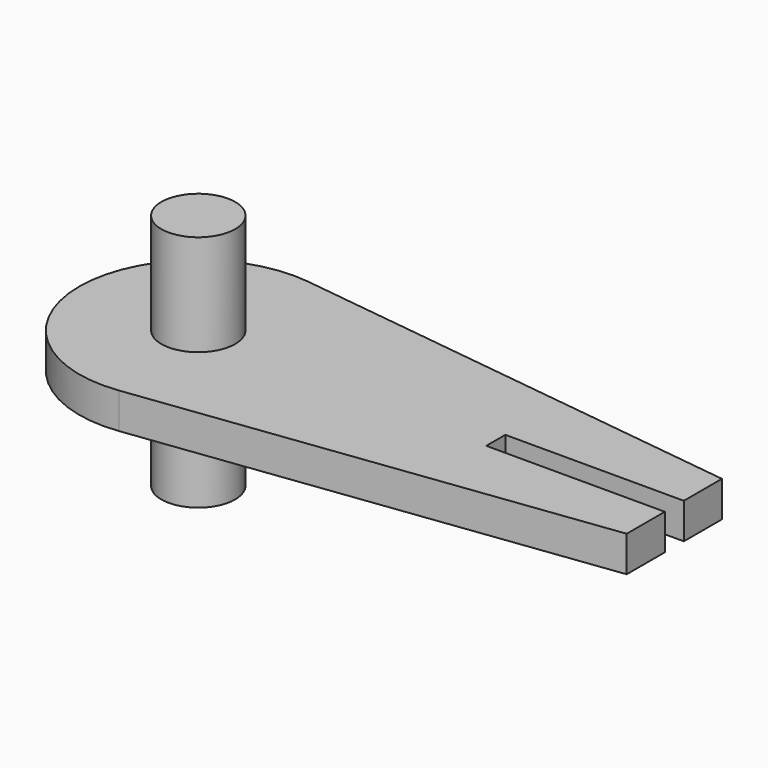
from build123d import *

# Parameters (mm, degrees)
F0_R     = 3.1
F1_DEPTH = 10
F2_DEPTH = 1.5
F3_W     = 15
F3_H     = 2
F4_DEPTH = 11.501


# Not quite as in the source:
# - a feature names something its author has since deleted; it is built from what else it names


with BuildPart() as f1:
    # F0 (on Top) → F1 (new body, symmetric)
    with BuildSketch(Plane.XY):
        Circle(F0_R)
    extrude(amount=F1_DEPTH, both=True)

    # F0 (on Top) → F2 (join, symmetric)
    with BuildSketch(Plane.XY):
        with BuildLine():
            ThreePointArc((1.2599617485, -9.9203072731), (7.5033198481, -6.6106120184), (10, 0))
            ThreePointArc((10, 0), (7.503319686, 6.6106122023), (1.2599612621, 9.9203073349))
            ThreePointArc((1.2599612621, 9.9203073349), (-10, -2.451e-07), (1.2599617485, -9.9203072731))
        make_face()
        Circle(F0_R, mode=Mode.SUBTRACT)
        with BuildLine():
            ThreePointArc((1.2599612621, 9.9203073349), (7.503319686, 6.6106122023), (10, 0))
            ThreePointArc((10, 0), (7.5033198481, -6.6106120184), (1.2599617485, -9.9203072731))
            Line((1.2599617485, -9.9203072731), (40, -5))
            Line((40, -5), (40, 5))
            Line((40, 5), (1.2599612621, 9.9203073349))
        make_face()
    extrude(amount=F2_DEPTH, both=True)

    # F3 (on face) → F4 (cut, through all)
    with BuildSketch(Plane.XY.offset(1.5)):
        with Locations((32.5, 0)):
            Rectangle(F3_W, F3_H)
    extrude(amount=-F4_DEPTH, mode=Mode.SUBTRACT)


solid = f1.part
